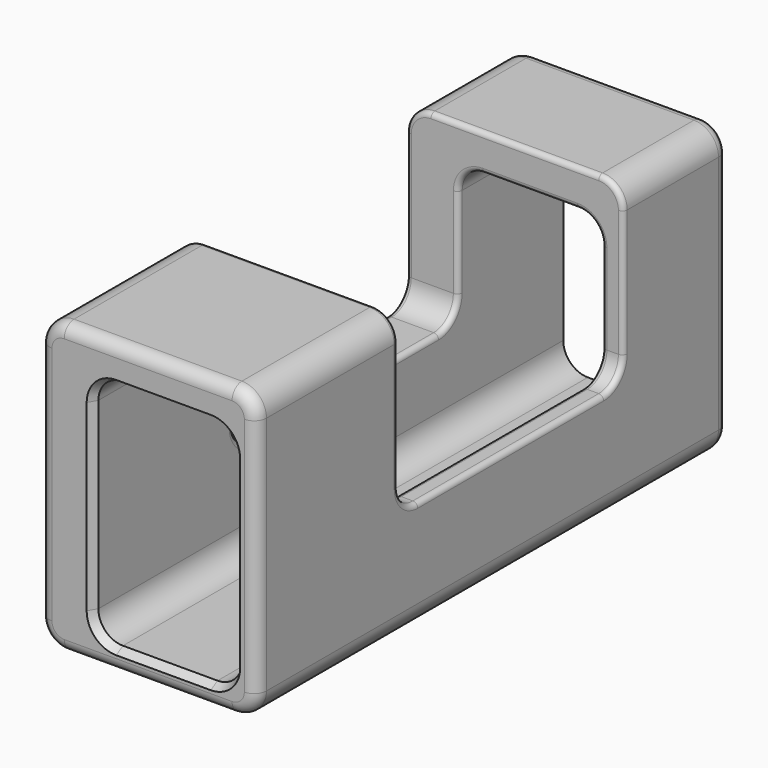
from build123d import *

# Parameters (mm, degrees)
F0_W      = 224.2983728647
F0_H      = 299.0915328264
F0_W_2    = 148.617759347
F0_H_2    = 240.4369190335
F1_DEPTH  = 609.6
F2_R      = 25.4
F3_R      = 25.4
F4_R      = 12.7
F5_R      = 12.7
F6_W      = 291.0227105021
F6_H      = 387.5585496426
F7_DEPTH  = 1050
F8_R      = 25.4
F9_R      = 5.08
F10_SIZE2 = 8.7988181024
F10_SIZE  = 5.08


# Not quite as in the source:
# - an extrude ends at something that could not be found from the text; its depth is read off the source's solid


with BuildPart() as f1:
    # F0 (on Front) → F1 (new body)
    with BuildSketch(Plane.XZ):
        with Locations((151.1405035853, 32.3162451386)):
            Rectangle(F0_W, F0_H)
        with Locations((166.9542267919, 23.8901861012)):
            Rectangle(F0_W_2, F0_H_2, mode=Mode.SUBTRACT)
    extrude(amount=F1_DEPTH)

    # F2
    f2_edges = [f1.edges().sort_by_distance(p)[0] for p in [
        (92.645347, -304.8, -96.328273),
        (241.263106, -304.8, -96.328273),
        (92.645347, -304.8, 144.108646),
        (241.263106, -304.8, 144.108646),
    ]]
    fillet(f2_edges, radius=F2_R)

    # F3
    f3_edges = [f1.edges().sort_by_distance(p)[0] for p in [
        (263.28969, -304.8, 181.862012),
        (38.991317, -304.8, 181.862012),
        (263.28969, -304.8, -117.229521),
        (38.991317, -304.8, -117.229521),
    ]]
    fillet(f3_edges, radius=F3_R)

    # F4
    f4_edges = [f1.edges().sort_by_distance(p)[0] for p in [
        (151.140504, -609.6, 181.862012),
    ]]
    fillet(f4_edges, radius=F4_R)

    # F5
    f5_edges = [f1.edges().sort_by_distance(p)[0] for p in [
        (151.140504, 0, 181.862012),
        (38.991317, 0, 32.316245),
        (46.430805, 0, 174.422524),
        (46.430805, 0, -109.790034),
        (151.140504, 0, -117.229521),
        (255.850202, 0, 174.422524),
        (255.850202, 0, -109.790034),
        (263.28969, 0, 32.316245),
    ]]
    fillet(f5_edges, radius=F5_R)

    # F6 (on face) → F7 (cut, through all)
    with BuildSketch(Plane.YZ.offset(263.2896900177)):
        with Locations((-281.2300659716, 193.7792748213)):
            Rectangle(F6_W, F6_H)
    extrude(amount=-F7_DEPTH, mode=Mode.SUBTRACT)

    # F8
    f8_edges = [f1.edges().sort_by_distance(p)[0] for p in [
        (65.818332, -135.718711, 0),
        (252.276398, -135.718711, 0),
        (65.818332, -426.741421, 0),
        (252.276398, -426.741421, 0),
    ]]
    fillet(f8_edges, radius=F8_R)

    # F9
    f9_edges = [f1.edges().sort_by_distance(p)[0] for p in [
        (92.645347, -281.230066, 0),
        (38.991317, -426.741421, 90.931006),
        (38.991317, -419.301933, 7.439488),
        (38.991317, -281.230066, 0),
        (38.991317, -143.158198, 7.439488),
        (38.991317, -135.718711, 90.931006),
        (263.28969, -426.741421, 90.931006),
        (255.850202, -426.741421, 174.422524),
        (241.263106, -426.741421, 72.054323),
        (151.140504, -426.741421, 181.862012),
        (233.823619, -426.741421, 136.669158),
        (46.430805, -426.741421, 174.422524),
        (166.954227, -426.741421, 144.108646),
        (100.084835, -426.741421, 136.669158),
        (92.645347, -426.741421, 72.054323),
        (92.645347, -419.301933, 7.439488),
        (92.645347, -143.158198, 7.439488),
        (263.28969, -135.718711, 90.931006),
        (255.850202, -135.718711, 174.422524),
        (241.263106, -135.718711, 72.054323),
        (151.140504, -135.718711, 181.862012),
        (233.823619, -135.718711, 136.669158),
        (46.430805, -135.718711, 174.422524),
        (166.954227, -135.718711, 144.108646),
        (100.084835, -135.718711, 136.669158),
        (92.645347, -135.718711, 72.054323),
        (263.28969, -143.158198, 7.439488),
        (263.28969, -281.230066, 0),
        (263.28969, -419.301933, 7.439488),
        (241.263106, -419.301933, 7.439488),
        (241.263106, -281.230066, 0),
        (241.263106, -143.158198, 7.439488),
    ]]
    fillet(f9_edges, radius=F9_R)

    # F10
    f10_edges = [f1.edges().sort_by_distance(p)[0] for p in [
        (166.954227, -609.6, -96.328273),
    ]]
    f10_side = f1.faces().sort_by_distance((151.140504, -609.6, 165.778705))[0]
    chamfer(f10_edges, length=F10_SIZE, length2=F10_SIZE2, reference=f10_side)


solid = f1.part
